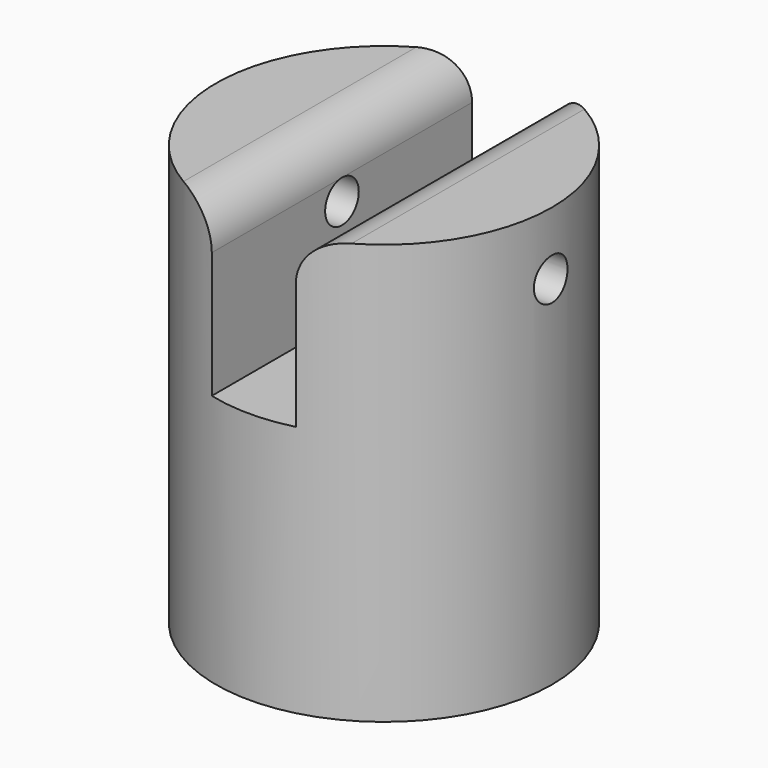
from build123d import *

# Parameters (mm, degrees)
F0_R     = 8
F1_DEPTH = 10
F2_W     = 4
F2_H     = 20
F3_DEPTH = 8
F4_R     = 1
F5_DEPTH = 12.5
F6_R     = 1.99999


# Not quite as in the source:
# - a fillet or chamfer is up to 0.001 mm smaller than in the source, because OpenCascade refuses the exact size


with BuildPart() as f1:
    # F0 (on Top) → F1 (new body, symmetric)
    with BuildSketch(Plane.XY):
        Circle(F0_R)
    extrude(amount=F1_DEPTH, both=True)

    # F2 (on face) → F3 (cut)
    with BuildSketch(Plane.XY.offset(10)):
        Rectangle(F2_W, F2_H)
    extrude(amount=-F3_DEPTH, mode=Mode.SUBTRACT)

    # F4 (on Right) → F5 (cut, symmetric)
    with BuildSketch(Plane.YZ):
        with Locations((0, 7)):
            Circle(F4_R)
    extrude(amount=F5_DEPTH, both=True, mode=Mode.SUBTRACT)

    # F6 (radius 2 in the source; OpenCascade refuses exactly that, so slightly less here)
    f6_edges = [f1.edges().sort_by_distance(p)[0] for p in [
        (-2, 0, 10),
        (2, 0, 10),
    ]]
    fillet(f6_edges, radius=F6_R)


solid = f1.part
